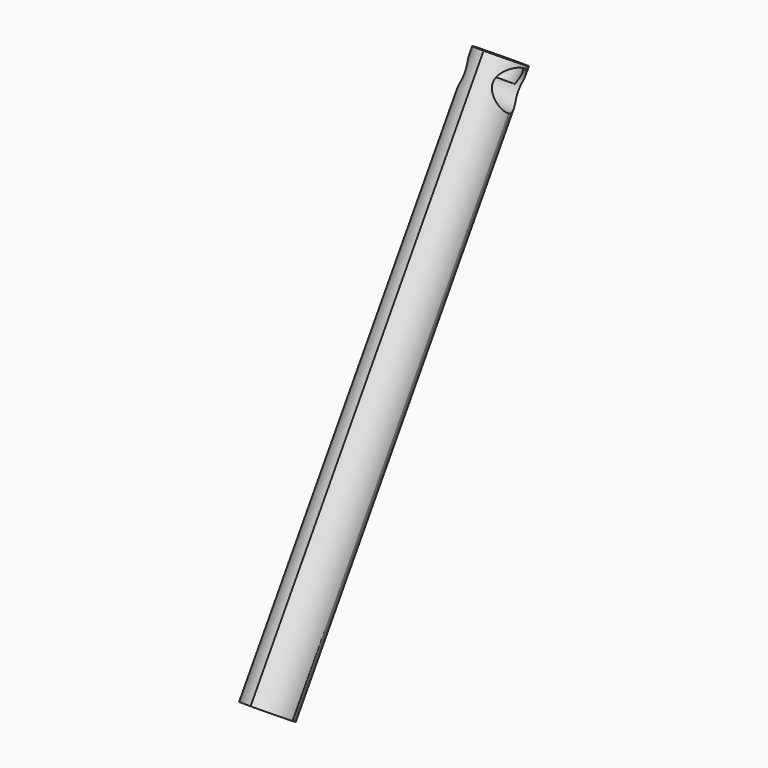
from build123d import *

# Parameters (mm, degrees)
F0_R        = 13.97
F1_DEPTH    = 19.05
F2_T1_DEPTH = 520.7
F2_T3_DEPTH = 520.7
F3_R        = 15.24
F4_DEPTH    = 12.7


# Not quite as in the source:
# - a fillet or chamfer that OpenCascade refuses, or shapes differently, is made with other operations: its cross-section is extruded or revolved along the edge and cut away or added


with BuildPart() as f1:
    # F0 (on Right) → F1 (new body, symmetric)
    with BuildSketch(Plane.YZ):
        Polygon((143.2134641072, 335.1731732972), (111.0520780853, 355.6), (-106.8340734116, 12.545215766), (-74.6726873897, -7.8816109369), align=None)
        with Locations((118.576942247, 332.0826940597)):
            Circle(F0_R, mode=Mode.SUBTRACT)
    extrude(amount=F1_DEPTH, both=True)

    # F2: fillet of radius 22.86 on 4 edges, made by hand

    # F2_s2 → F2_t1 (cut)
    with BuildSketch(Plane(origin=(0, 223.4952640736, 351.8861527791), x_dir=(1, 0, 0), z_dir=(0, -0.5361371838, -0.8441308667))):
        with BuildLine():
            ThreePointArc((19.05, 74.0478956349), (12.3544610179, 90.2123566528), (-3.81, 96.9078956349))
            Line((-3.81, 96.9078956349), (19.05, 96.9078956349))
            Line((19.05, 96.9078956349), (19.05, 74.0478956349))
        make_face()
        with BuildLine():
            ThreePointArc((3.81, 96.9078956349), (-12.3544610179, 90.2123566528), (-19.05, 74.0478956349))
            Line((-19.05, 74.0478956349), (-19.05, 96.9078956349))
            Line((-19.05, 96.9078956349), (3.81, 96.9078956349))
        make_face()
    extrude(amount=F2_T1_DEPTH, mode=Mode.SUBTRACT)

    # F2_s4 → F2_t3 (cut)
    with BuildSketch(Plane(origin=(0, -55.6713675318, -87.6527895208), x_dir=(1, 0, 0), z_dir=(0, 0.5361371838, 0.8441308667))):
        with BuildLine():
            ThreePointArc((-3.81, -58.8078956349), (12.3544610179, -65.5034346169), (19.05, -81.6678956349))
            Line((19.05, -81.6678956349), (19.05, -58.8078956349))
            Line((19.05, -58.8078956349), (-3.81, -58.8078956349))
        make_face()
        with BuildLine():
            ThreePointArc((3.81, -58.8078956349), (-12.3544610179, -65.5034346169), (-19.05, -81.6678956349))
            Line((-19.05, -81.6678956349), (-19.05, -58.8078956349))
            Line((-19.05, -58.8078956349), (3.81, -58.8078956349))
        make_face()
    extrude(amount=F2_T3_DEPTH, mode=Mode.SUBTRACT)

    # F3 (on face) → F4 (cut, symmetric)
    with BuildSketch(Plane(origin=(0, 192.8550240193, 303.6440737462), x_dir=(1, 0, 0), z_dir=(0, 0.5361371838, 0.8441308667))):
        with Locations((0, -77.8578956349)):
            Circle(F3_R)
    extrude(amount=F4_DEPTH, both=True, mode=Mode.SUBTRACT)


solid = f1.part
